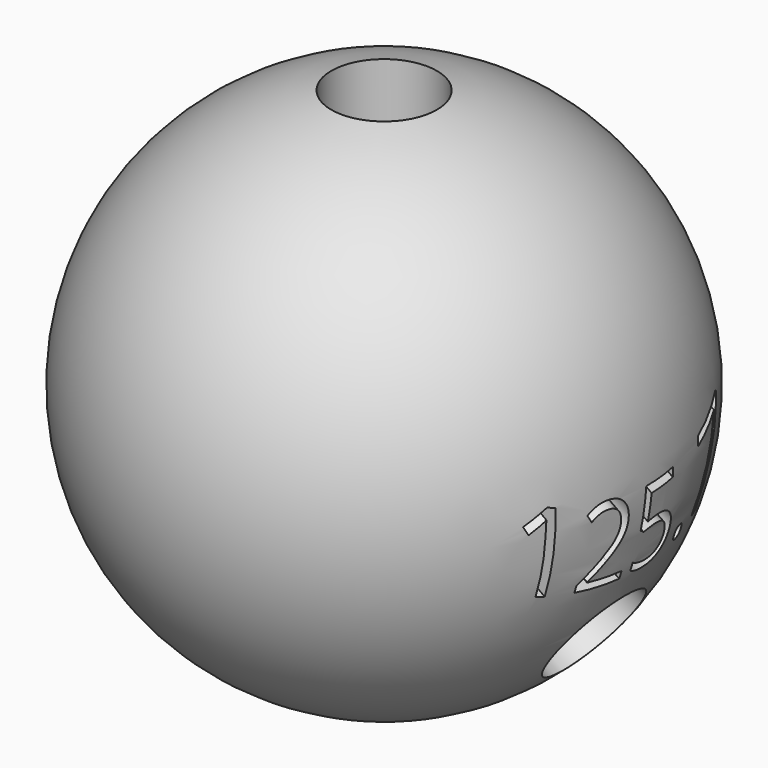
from build123d import *

# Parameters (mm, degrees)
F4_R          = 3.175
F5_DEPTH      = 50.8
F7_ANGLE      = 125.7
F8_ANGLE      = -125.7
F10_TEXT_SIZE = 6.1190053303
F11_DEPTH     = 23.4696
F13_TEXT_SIZE = 4.9194987191
F14_DEPTH     = 20.9804


# Not quite as in the source:
# - Text() gives the source's letters only with a copy of the font that has no kerning and outlines rounded to 1/6400 em; it was checked with that copy


with BuildPart() as f2:
    # F0 (on Front) → F2 (revolve)
    with BuildSketch(Plane.XZ):
        with BuildLine():
            Line((0, -15.875), (0, 15.875))
            ThreePointArc((0, 15.875), (-15.875, 0), (0, -15.875))
        make_face()
    revolve(axis=Axis((0, 0, 0), (0, 0, 1)))

    # F10 (on offset) → F11 (cut)
    with BuildSketch(Plane(origin=(25.7836519788, 0, -18.5274334606), x_dir=(0, 1, 0), z_dir=(0.8120835269, 0, -0.5835412114))):
        with Locations((-7.7853850089, 4.7376127914)):
            Text('125.7', F10_TEXT_SIZE, font='Open Sans', text_align=(TextAlign.LEFT, TextAlign.BOTTOM))
    extrude(amount=-F11_DEPTH, mode=Mode.SUBTRACT)

    # F13 (on offset) → F14 (cut)
    with BuildSketch(Plane(origin=(-25.7836519788, 0, -18.5274334606), x_dir=(0, -1, 0), z_dir=(-0.8120835269, 0, -0.5835412114))):
        with Locations((-6.1140940525, 5.5598984472)):
            Text('125.7', F13_TEXT_SIZE, font='Open Sans', text_align=(TextAlign.LEFT, TextAlign.BOTTOM))
    extrude(amount=-F14_DEPTH, mode=Mode.SUBTRACT)


with BuildPart() as f5:
    # F4 (on offset) → F5 (new body)
    with BuildSketch(Plane.XY.offset(6.35)):
        Circle(F4_R)
    extrude(amount=F5_DEPTH)


with BuildPart() as f7_1:
    # F7: copy of F5
    add(f5.part.rotate(Axis((0, -37.4240316451, 0), (0, -1, 0)), F7_ANGLE))


with BuildPart() as f8_1:
    # F8: copy of F5
    add(f5.part.rotate(Axis((0, -37.4240316451, 0), (0, -1, 0)), F8_ANGLE))


with BuildPart() as f2_1:
    add(f2.part)

    # F15: cut F5, F7_1, F8_1
    add(f5.part, mode=Mode.SUBTRACT)
    add(f7_1.part, mode=Mode.SUBTRACT)
    add(f8_1.part, mode=Mode.SUBTRACT)


solid = f2_1.part
